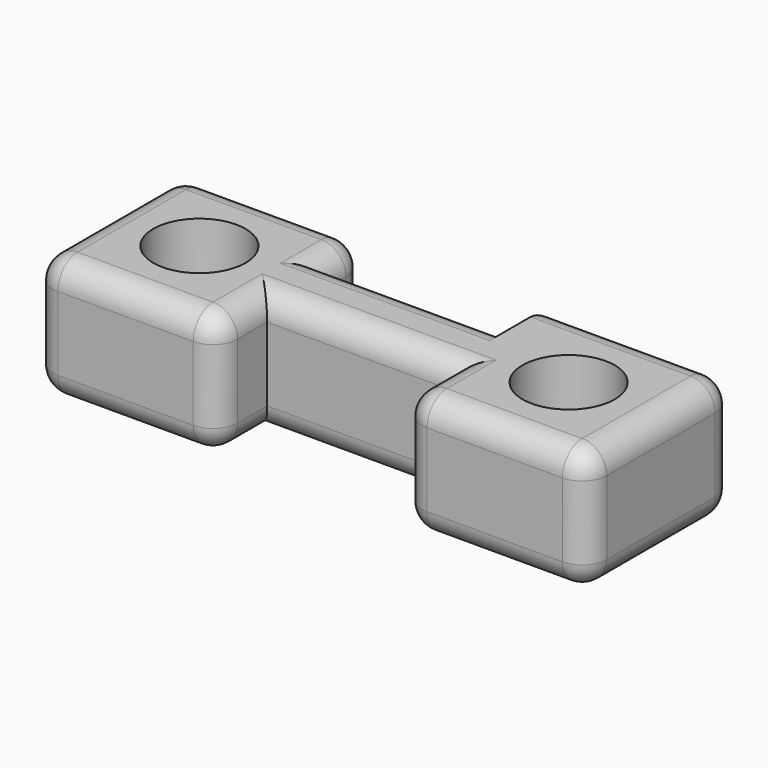
from build123d import *

# Parameters (mm, degrees)
F0_R         = 9.525
F0_W         = 38.1
F0_H         = 14.8362964392
F1_DEPTH     = 25.4
F2_R         = 5.08
F3_T1_DEPTH  = 15.24
F3_S5_W      = 5.08
F3_S5_H      = 5.08
F3_T6_DEPTH  = 5.08
F3_S11_W     = 5.08
F3_S11_H     = 5.08
F3_T12_DEPTH = 5.08
F3_S17_W     = 5.08
F3_S17_H     = 5.08
F3_T18_DEPTH = 5.08
F3_S23_W     = 5.08
F3_S23_H     = 5.08
F3_T24_DEPTH = 5.08


# Not quite as in the source:
# - a fillet or chamfer that OpenCascade refuses, or shapes differently, is made with other operations: its cross-section is extruded or revolved along the edge and cut away or added


with BuildPart() as f1:
    # F0 (on Top) → F1 (new body)
    with BuildSketch(Plane.XY):
        Polygon((-105.0124109644, 7.0207449608), (-66.9124109644, 7.0207449608), (-66.9124109644, 19.73756589), (-66.9124109644, 34.5738623291), (-66.9124109644, 45.1207449608), (-105.0124109644, 45.1207449608), align=None)
        with Locations((-85.9624109644, 26.0707449608)):
            Circle(F0_R, mode=Mode.SUBTRACT)
        with Locations((-47.8624109644, 27.1557141095)):
            Rectangle(F0_W, F0_H)
        Polygon((-28.8124109644, 34.5738623291), (-28.8124109644, 19.73756589), (-28.8124109644, 7.0207449608), (9.2875890356, 7.0207449608), (9.2875890356, 45.1207449608), (-28.8124109644, 45.1207449608), align=None)
        with Locations((-9.7624109644, 26.0707449608)):
            Circle(F0_R, mode=Mode.SUBTRACT)
    extrude(amount=F1_DEPTH)

    # F2
    f2_edges = [f1.edges().sort_by_distance(p)[0] for p in [
        (-85.962411, 45.120745, 25.4),
        (-85.962411, 45.120745, 0),
        (-105.012411, 45.120745, 12.7),
        (-105.012411, 26.070745, 0),
        (-105.012411, 26.070745, 25.4),
        (-85.962411, 7.020745, 25.4),
        (-47.862411, 19.737566, 25.4),
        (-47.862411, 34.573862, 25.4),
        (-66.912411, 39.847304, 25.4),
        (-66.912411, 13.379155, 25.4),
        (-28.812411, 13.379155, 25.4),
        (-9.762411, 7.020745, 25.4),
        (9.287589, 26.070745, 25.4),
        (-9.762411, 45.120745, 25.4),
        (9.287589, 7.020745, 12.7),
        (9.287589, 45.120745, 12.7),
        (9.287589, 26.070745, 0),
        (-47.862411, 19.737566, 0),
        (-66.912411, 13.379155, 0),
        (-66.912411, 7.020745, 12.7),
        (-28.812411, 7.020745, 12.7),
        (-85.962411, 7.020745, 0),
        (-47.862411, 34.573862, 0),
        (-9.762411, 45.120745, 0),
        (-28.812411, 45.120745, 12.7),
        (-28.812411, 39.847304, 0),
        (-66.912411, 39.847304, 0),
        (-9.762411, 7.020745, 0),
        (-28.812411, 13.379155, 0),
    ]]
    fillet(f2_edges, radius=F2_R)

    # F3: fillet of radius 5.08 on 2 edges, made by hand

    # F3_s2 → F3_t1 (cut)
    with BuildSketch(Plane.XY.offset(5.08)):
        with BuildLine():
            ThreePointArc((-71.9924109644, 45.1207449608), (-68.4003085159, 43.6328474092), (-66.9124109644, 40.0407449608))
            Line((-66.9124109644, 40.0407449608), (-66.9124109644, 45.1207449608))
            Line((-66.9124109644, 45.1207449608), (-71.9924109644, 45.1207449608))
        make_face()
        with BuildLine():
            ThreePointArc((-105.0124109644, 12.1007449608), (-103.5245134128, 8.5086425123), (-99.9324109644, 7.0207449608))
            Line((-99.9324109644, 7.0207449608), (-105.0124109644, 7.0207449608))
            Line((-105.0124109644, 7.0207449608), (-105.0124109644, 12.1007449608))
        make_face()
    extrude(amount=F3_T1_DEPTH, mode=Mode.SUBTRACT)


with BuildPart() as f3_tool4:
    # F3_s5 → F3_t6 (new body)
    with BuildSketch(Plane.YZ.offset(-99.9324109644)):
        with Locations((9.5607449608, 2.54)):
            Rectangle(F3_S5_W, F3_S5_H)
    extrude(amount=-F3_T6_DEPTH)

    # F3_s7 → F3_t8 (revolve, cut)
    with BuildSketch(Plane(origin=(-99.9324109644, 12.1007449608, 5.08), x_dir=(0, 0.7071067812, 0.7071067812), z_dir=(0, -0.7071067812, 0.7071067812))):
        with BuildLine():
            ThreePointArc((0, -5.08), (5.08, 0), (0, 5.08))
            Line((0, 5.08), (0, -5.08))
        make_face()
    revolve(axis=Axis((-99.9324109644, 12.1007449608, 5.08), (-1, 0, 0)), mode=Mode.SUBTRACT)


with BuildPart() as f1_1:
    add(f1.part)

    # F3_t3: cut F3_tool4
    add(f3_tool4.part, mode=Mode.SUBTRACT)


with BuildPart() as f3_tool10:
    # F3_s11 → F3_t12 (new body)
    with BuildSketch(Plane.YZ.offset(-99.9324109644)):
        with Locations((9.5607449608, 22.86)):
            Rectangle(F3_S11_W, F3_S11_H)
    extrude(amount=-F3_T12_DEPTH)

    # F3_s13 → F3_t14 (revolve, cut)
    with BuildSketch(Plane(origin=(-99.9324109644, 12.1007449608, 20.32), x_dir=(0, 0.7071067812, -0.7071067812), z_dir=(0, 0.7071067812, 0.7071067812))):
        with BuildLine():
            ThreePointArc((0, -5.08), (5.08, 0), (0, 5.08))
            Line((0, 5.08), (0, -5.08))
        make_face()
    revolve(axis=Axis((-99.9324109644, 12.1007449608, 20.32), (-1, 0, 0)), mode=Mode.SUBTRACT)


with BuildPart() as f1_2:
    add(f1_1.part)

    # F3_t9: cut F3_tool10
    add(f3_tool10.part, mode=Mode.SUBTRACT)


with BuildPart() as f3_tool16:
    # F3_s17 → F3_t18 (new body)
    with BuildSketch(Plane.XZ.offset(-40.0407449608)):
        with Locations((-69.4524109644, 2.54)):
            Rectangle(F3_S17_W, F3_S17_H)
    extrude(amount=-F3_T18_DEPTH)

    # F3_s19 → F3_t20 (revolve, cut)
    with BuildSketch(Plane(origin=(-71.9924109644, 40.0407449608, 5.08), x_dir=(-0.7071067812, 0, 0.7071067812), z_dir=(-0.7071067812, 0, -0.7071067812))):
        with BuildLine():
            ThreePointArc((0, -5.08), (5.08, 0), (0, 5.08))
            Line((0, 5.08), (0, -5.08))
        make_face()
    revolve(axis=Axis((-71.9924109644, 40.0407449608, 5.08), (0, 1, 0)), mode=Mode.SUBTRACT)


with BuildPart() as f1_3:
    add(f1_2.part)

    # F3_t15: cut F3_tool16
    add(f3_tool16.part, mode=Mode.SUBTRACT)


with BuildPart() as f3_tool22:
    # F3_s23 → F3_t24 (new body)
    with BuildSketch(Plane.XZ.offset(-40.0407449608)):
        with Locations((-69.4524109644, 22.86)):
            Rectangle(F3_S23_W, F3_S23_H)
    extrude(amount=-F3_T24_DEPTH)

    # F3_s25 → F3_t26 (revolve, cut)
    with BuildSketch(Plane(origin=(-71.9924109644, 40.0407449608, 20.32), x_dir=(-0.7071067812, 0, -0.7071067812), z_dir=(0.7071067812, 0, -0.7071067812))):
        with BuildLine():
            ThreePointArc((0, -5.08), (5.08, 0), (0, 5.08))
            Line((0, 5.08), (0, -5.08))
        make_face()
    revolve(axis=Axis((-71.9924109644, 40.0407449608, 20.32), (0, 1, 0)), mode=Mode.SUBTRACT)


with BuildPart() as f1_4:
    add(f1_3.part)

    # F3_t21: cut F3_tool22
    add(f3_tool22.part, mode=Mode.SUBTRACT)


solid = f1_4.part
